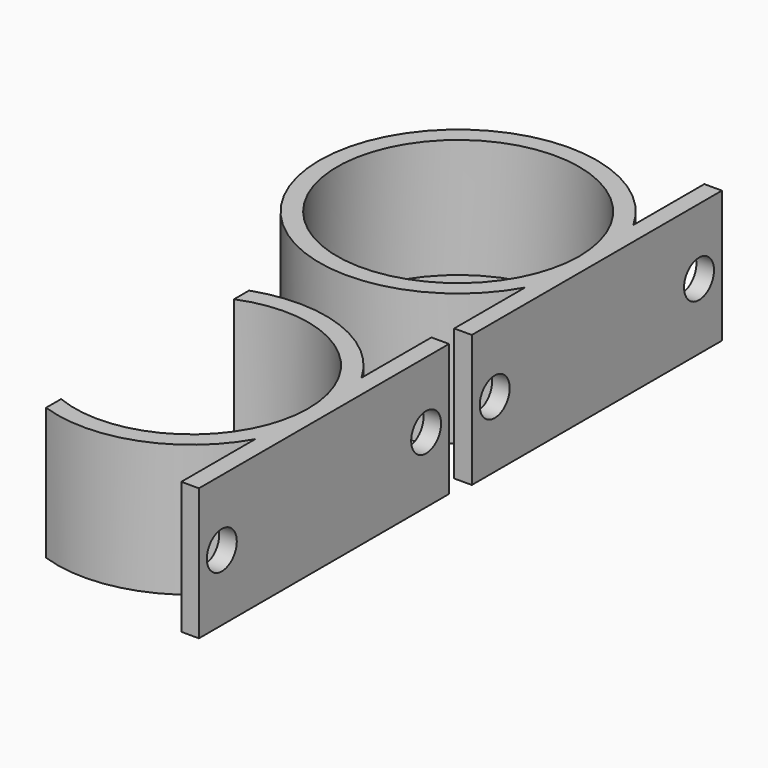
from build123d import *

# Parameters (mm, degrees)
F0_R      = 31.5
F0_R_2    = 27.5
F1_DEPTH  = 30
F2_R      = 31.5
F2_R_2    = 27.5
F3_DEPTH  = 3
F5_DEPTH  = 30
F6_R      = 4.25
F7_DEPTH  = 5
F9_DEPTH  = 30
F10_R     = 4.25
F11_DEPTH = 5


# Not quite as in the source:
# - a feature names something its author has since deleted; it is built from what else it names


with BuildPart() as f1:
    # F0 (on Top) → F1 (new body)
    with BuildSketch(Plane.XY):
        Circle(F0_R)
        Circle(F0_R_2, mode=Mode.SUBTRACT)
    extrude(amount=F1_DEPTH)

    # F2 (on face) → F3 (join)
    with BuildSketch(Plane(origin=(0, 0, 0), x_dir=(1, 0, 0), z_dir=(0, 0, -1))):
        Circle(F2_R)
        Circle(F2_R_2, mode=Mode.SUBTRACT)
        Circle(F2_R_2)
    extrude(amount=-F3_DEPTH)

    # F4 (on face) → F5 (join)
    with BuildSketch(Plane.XY.offset(30)):
        with BuildLine():
            Line((27.5, 35.5), (27.5, 15.3622914957))
            ThreePointArc((27.5, 15.3622914957), (30.4836021494, 7.9372539332), (31.5, 0))
            Line((31.5, 0), (31.5, 35.5))
            Line((31.5, 35.5), (27.5, 35.5))
        make_face()
        with BuildLine():
            ThreePointArc((31.5, 0), (30.4836021494, -7.9372539332), (27.5, -15.3622914957))
            Line((27.5, -15.3622914957), (27.5, -35.5))
            Line((27.5, -35.5), (31.5, -35.5))
            Line((31.5, -35.5), (31.5, 0))
        make_face()
    extrude(amount=-F5_DEPTH)

    # F6 (on face) → F7 (cut)
    with BuildSketch(Plane.YZ.offset(31.5)):
        with Locations((29, 15)):
            Circle(F6_R)
        with Locations((-29, 15)):
            Circle(F6_R)
    extrude(amount=-F7_DEPTH, mode=Mode.SUBTRACT)


with BuildPart() as f9:
    # F8 (on Top) → F9 (new body)
    with BuildSketch(Plane.XY):
        with BuildLine():
            Line((26.5, -76.2157712579), (26.5, -75.6643489003))
            ThreePointArc((26.5, -75.6643489003), (14.7859730826, -97.6558245216), (-10, -100.2051312839))
            Line((-10, -100.2051312839), (-10, -104.4784079688))
            ThreePointArc((-10, -104.4784079688), (10.7277036045, -104.2154675365), (26.5, -90.7640177709))
            Line((26.5, -90.7640177709), (26.5, -76.2157712579))
        make_face()
        with BuildLine():
            Line((26.5, -60.5646800298), (26.5, -75.6643489003))
            Line((26.5, -75.6643489003), (26.5, -76.2157712579))
            Line((26.5, -76.2157712579), (26.5, -90.7640177709))
            ThreePointArc((26.5, -90.7640177709), (29.4830459756, -83.4745985762), (30.5, -75.6643489003))
            ThreePointArc((30.5, -75.6643489003), (29.4830459756, -67.8540992244), (26.5, -60.5646800298))
        make_face()
        with BuildLine():
            ThreePointArc((-10, -51.1235665167), (14.7859730826, -53.6728732791), (26.5, -75.6643489003))
            Line((26.5, -75.6643489003), (26.5, -60.5646800298))
            ThreePointArc((26.5, -60.5646800298), (10.7277036045, -47.1132302642), (-10, -46.8502898319))
            Line((-10, -46.8502898319), (-10, -51.1235665167))
        make_face()
        with BuildLine():
            Line((26.5, -40.7157712579), (26.5, -60.5646800298))
            ThreePointArc((26.5, -60.5646800298), (29.4830459756, -67.8540992244), (30.5, -75.6643489003))
            Line((30.5, -75.6643489003), (30.5, -40.7157712579))
            Line((30.5, -40.7157712579), (26.5, -40.7157712579))
        make_face()
        with BuildLine():
            ThreePointArc((30.5, -75.6643489003), (29.4830459756, -83.4745985762), (26.5, -90.7640177709))
            Line((26.5, -90.7640177709), (26.5, -111.7157712579))
            Line((26.5, -111.7157712579), (30.5, -111.7157712579))
            Line((30.5, -111.7157712579), (30.5, -75.6643489003))
        make_face()
    extrude(amount=F9_DEPTH)

    # F10 (on face) → F11 (cut)
    with BuildSketch(Plane.YZ.offset(30.5)):
        with Locations((-105.2157712579, 15)):
            Circle(F10_R)
        with Locations((-47.2157712579, 15)):
            Circle(F10_R)
    extrude(amount=-F11_DEPTH, mode=Mode.SUBTRACT)


solid = Compound([f1.part, f9.part])
